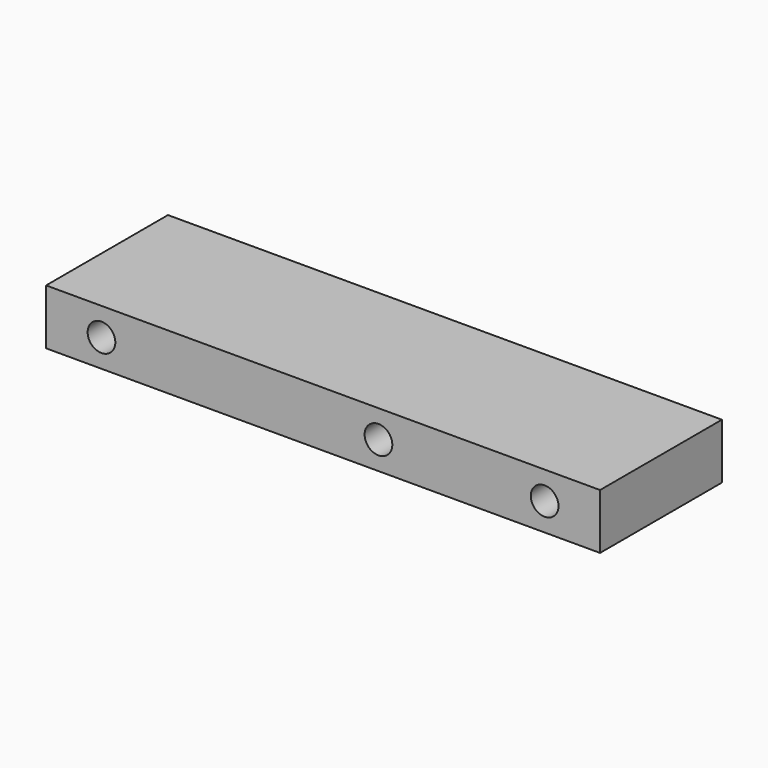
from build123d import *

# Parameters (mm, degrees)
F0_W     = 127
F0_H     = 12.7
F1_DEPTH = 34.925
F2_R     = 3.175
F3_DEPTH = 34.925


# Not quite as in the source:
# - a feature names something its author has since deleted; it is built from what else it names


with BuildPart() as f1:
    # F0 (on Front) → F1 (new body)
    with BuildSketch(Plane.XZ):
        with Locations((-31.0538060308, 35.6538111673)):
            Rectangle(F0_W, F0_H)
    extrude(amount=F1_DEPTH)

    # F2 (on face) → F3 (cut)
    with BuildSketch(Plane.XZ.offset(34.925)):
        with Locations((-81.8538060308, 35.6538111673)):
            Circle(F2_R)
        with Locations((-18.3538060308, 35.6538111673)):
            Circle(F2_R)
        with Locations((19.7461939692, 35.6538111673)):
            Circle(F2_R)
    extrude(amount=-F3_DEPTH, mode=Mode.SUBTRACT)


solid = f1.part
